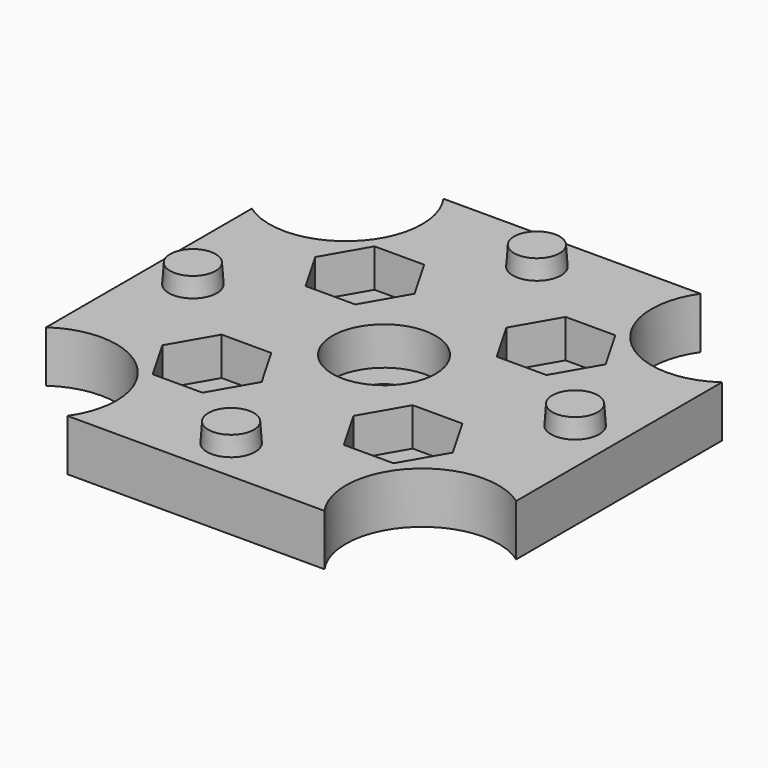
from build123d import *

# Parameters (mm, degrees)
F0_R       = 3.2004
F0_R_2     = 6.858
F1_DEPTH   = 6.8326
F2_DEPTH   = 9.3726
F3_R       = 3.2004
F3_R_2     = 6.858
F4_DEPTH   = 5.08
F5_SIZE2   = 2.53999
F5_SIZE    = 0.17779
F5_2_SIZE2 = 2.53999
F5_2_SIZE  = 0.17779
F5_3_SIZE2 = 2.53999
F5_3_SIZE  = 0.17779
F5_4_SIZE2 = 2.53999
F5_4_SIZE  = 0.17779


# Not quite as in the source:
# - a fillet or chamfer is up to 0.001 mm smaller than in the source, because OpenCascade refuses the exact size


with BuildPart() as f1:
    # F0 (on Top) → F1 (new body)
    with BuildSketch(Plane.XY):
        with BuildLine():
            ThreePointArc((-31.242, -17.0875613686), (-20.7164714157, -16.3838944106), (-15.24, -25.4))
            ThreePointArc((-15.24, -25.4), (-15.712895776, -28.4635945803), (-17.0875613686, -31.242))
            Line((-17.0875613686, -31.242), (17.0875613686, -31.242))
            ThreePointArc((17.0875613686, -31.242), (18.2157951031, -18.2157951031), (31.242, -17.0875613686))
            Line((31.242, -17.0875613686), (31.242, 17.0875613686))
            ThreePointArc((31.242, 17.0875613686), (18.2157951031, 18.2157951031), (17.0875613686, 31.242))
            Line((17.0875613686, 31.242), (-17.0875613686, 31.242))
            ThreePointArc((-17.0875613686, 31.242), (-18.2157951031, 18.2157951031), (-31.242, 17.0875613686))
            Line((-31.242, 17.0875613686), (-31.242, -17.0875613686))
        make_face()
        with Locations((0, -25.4)):
            Circle(F0_R, mode=Mode.SUBTRACT)
        with Locations((-25.4, 0)):
            Circle(F0_R, mode=Mode.SUBTRACT)
        with Locations((-12.7, -12.7)):
            Circle(F0_R, mode=Mode.SUBTRACT)
        Circle(F0_R_2, mode=Mode.SUBTRACT)
        with Locations((12.7, -12.7)):
            Circle(F0_R, mode=Mode.SUBTRACT)
        with Locations((25.4, 0)):
            Circle(F0_R, mode=Mode.SUBTRACT)
        with Locations((-12.7, 12.7)):
            Circle(F0_R, mode=Mode.SUBTRACT)
        with Locations((0, 25.4)):
            Circle(F0_R, mode=Mode.SUBTRACT)
        with Locations((12.7, 12.7)):
            Circle(F0_R, mode=Mode.SUBTRACT)
        Circle(F0_R_2)
        Circle(F0_R, mode=Mode.SUBTRACT)
    extrude(amount=F1_DEPTH)

    # F0 (on Top) → F2 (join)
    with BuildSketch(Plane.XY):
        with Locations((-25.4, 0)):
            Circle(F0_R)
        with Locations((0, -25.4)):
            Circle(F0_R)
        with Locations((25.4, 0)):
            Circle(F0_R)
        with Locations((0, 25.4)):
            Circle(F0_R)
    extrude(amount=F2_DEPTH)

    # F3 (on face) → F4 (cut)
    with BuildSketch(Plane.XY.offset(6.8326)):
        Polygon((-9.398, 6.9807682334), (-6.096, 12.7), (-9.398, 18.4192317666), (-16.002, 18.4192317666), (-19.304, 12.7), (-16.002, 6.9807682334), align=None)
        with Locations((-12.7, 12.7)):
            Circle(F3_R, mode=Mode.SUBTRACT)
        Polygon((9.398, 18.4192317666), (6.096, 12.7), (9.398, 6.9807682334), (16.002, 6.9807682334), (19.304, 12.7), (16.002, 18.4192317666), align=None)
        with Locations((12.7, 12.7)):
            Circle(F3_R, mode=Mode.SUBTRACT)
        Polygon((-9.398, -18.4192317666), (-6.096, -12.7), (-9.398, -6.9807682334), (-16.002, -6.9807682334), (-19.304, -12.7), (-16.002, -18.4192317666), align=None)
        with Locations((-12.7, -12.7)):
            Circle(F3_R, mode=Mode.SUBTRACT)
        Polygon((9.398, -6.9807682334), (6.096, -12.7), (9.398, -18.4192317666), (16.002, -18.4192317666), (19.304, -12.7), (16.002, -6.9807682334), align=None)
        with Locations((12.7, -12.7)):
            Circle(F3_R, mode=Mode.SUBTRACT)
        Circle(F3_R_2)
        Circle(F3_R, mode=Mode.SUBTRACT)
    extrude(amount=-F4_DEPTH, mode=Mode.SUBTRACT)

    # F5 (size 0.1778 and 2.54 in the source; OpenCascade refuses exactly that, so slightly less here)
    f5_edges = [f1.edges().sort_by_distance(p)[0] for p in [
        (-28.6004, 0, 9.3726),
    ]]
    f5_side = f1.faces().sort_by_distance((-25.4, 0, 9.3726))[0]
    chamfer(f5_edges, length=F5_SIZE, length2=F5_SIZE2, reference=f5_side)

    # F5#2 (size 0.1778 and 2.54 in the source; OpenCascade refuses exactly that, so slightly less here)
    f5_2_edges = [f1.edges().sort_by_distance(p)[0] for p in [
        (-3.2004, 25.4, 9.3726),
    ]]
    f5_2_side = f1.faces().sort_by_distance((0, 25.4, 9.3726))[0]
    chamfer(f5_2_edges, length=F5_2_SIZE, length2=F5_2_SIZE2, reference=f5_2_side)

    # F5#3 (size 0.1778 and 2.54 in the source; OpenCascade refuses exactly that, so slightly less here)
    f5_3_edges = [f1.edges().sort_by_distance(p)[0] for p in [
        (22.1996, 0, 9.3726),
    ]]
    f5_3_side = f1.faces().sort_by_distance((25.4, 0, 9.3726))[0]
    chamfer(f5_3_edges, length=F5_3_SIZE, length2=F5_3_SIZE2, reference=f5_3_side)

    # F5#4 (size 0.1778 and 2.54 in the source; OpenCascade refuses exactly that, so slightly less here)
    f5_4_edges = [f1.edges().sort_by_distance(p)[0] for p in [
        (-3.2004, -25.4, 9.3726),
    ]]
    f5_4_side = f1.faces().sort_by_distance((0, -25.4, 9.3726))[0]
    chamfer(f5_4_edges, length=F5_4_SIZE, length2=F5_4_SIZE2, reference=f5_4_side)


solid = f1.part
